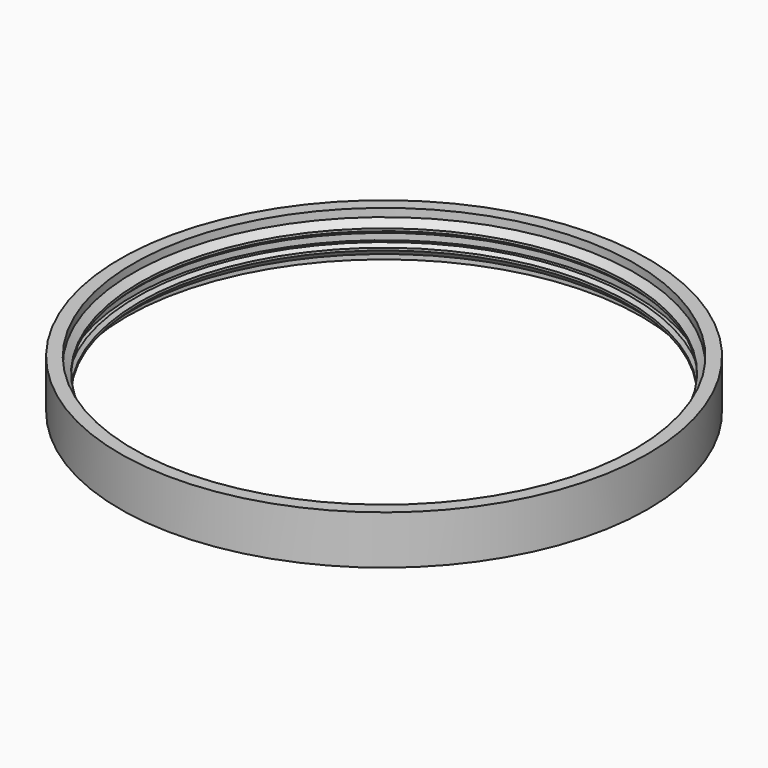
from build123d import *

# Parameters (mm, degrees)
F0_R      = 16.25
F1_DEPTH  = 1.5
F2_R      = 15.05
F3_DEPTH  = 3.001
F4_R      = 15.45
F5_DEPTH  = 0.25
F6_SIZE   = 0.2
F7_R      = 15.45
F8_DEPTH  = 0.5
F9_R      = 15.85
F10_DEPTH = 0.5
F11_SIZE  = 0.39999


# Not quite as in the source:
# - a fillet or chamfer is up to 0.001 mm smaller than in the source, because OpenCascade refuses the exact size


with BuildPart() as f1:
    # F0 (on Top) → F1 (new body, symmetric)
    with BuildSketch(Plane.XY):
        Circle(F0_R)
    extrude(amount=F1_DEPTH, both=True)

    # F2 (on face) → F3 (cut, through all)
    with BuildSketch(Plane.XY.offset(1.5)):
        Circle(F2_R)
    extrude(amount=-F3_DEPTH, mode=Mode.SUBTRACT)

    # F4 (on Top) → F5 (cut, symmetric)
    with BuildSketch(Plane.XY):
        Circle(F4_R)
    extrude(amount=F5_DEPTH, both=True, mode=Mode.SUBTRACT)

    # F6
    f6_edges = [f1.edges().sort_by_distance(p)[0] for p in [
        (-15.05, 0, 0.25),
        (-15.05, 0, -0.25),
    ]]
    chamfer(f6_edges, length=F6_SIZE)

    # F7 (on face) → F8 (cut)
    with BuildSketch(Plane.XY.offset(1.5)):
        Circle(F7_R)
    extrude(amount=-F8_DEPTH, mode=Mode.SUBTRACT)

    # F9 (on face) → F10 (cut)
    with BuildSketch(Plane(origin=(0, 0, -1.5), x_dir=(1, 0, 0), z_dir=(0, 0, -1))):
        Circle(F9_R)
    extrude(amount=-F10_DEPTH, mode=Mode.SUBTRACT)

    # F11 (size 0.4 in the source; OpenCascade refuses exactly that, so slightly less here)
    f11_edges = [f1.edges().sort_by_distance(p)[0] for p in [
        (-15.05, 0, 1),
        (-15.05, 0, -1),
    ]]
    chamfer(f11_edges, length=F11_SIZE)


solid = f1.part
